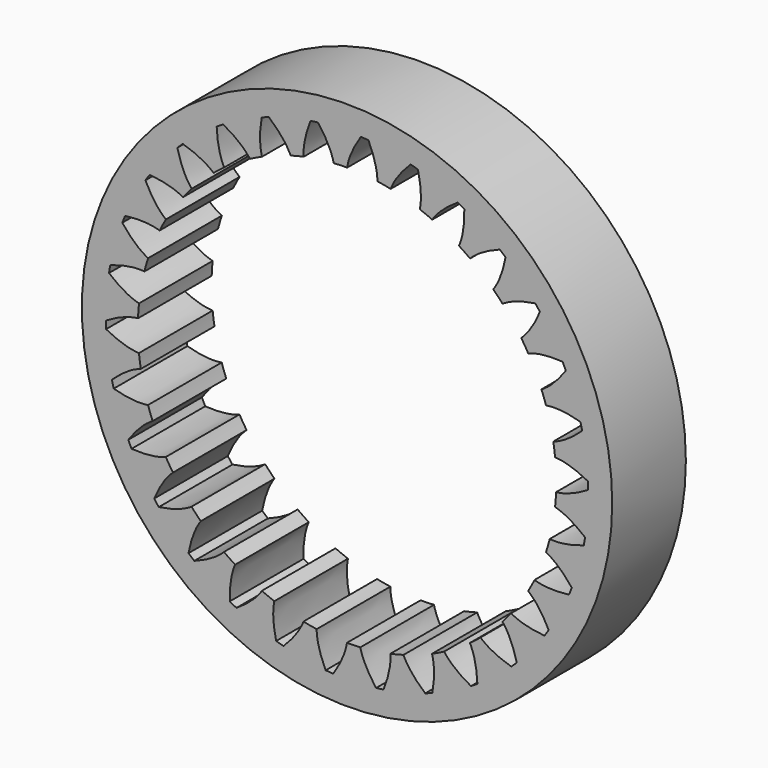
from build123d import *

# Parameters (mm, degrees)
F0_R            = 14.4
F1_DEPTH        = 5
F2_DEPTH        = 5
F2_COPIES_COUNT = 30


# Not quite as in the source:
# - a pattern or mirror of a feature is missing from the dataset's text; its kind, count and spacing are read off the source's solid


with BuildPart() as f1:
    # F0 (on Front) → F1 (new body)
    with BuildSketch(Plane.XZ):
        Circle(F0_R)
        with BuildLine():
            ThreePointArc((-1.576958744, 13.0047376413), (-0.4143593333, 13.0934451671), (0.7515226609, 13.078425505))
            ThreePointArc((0.7515226609, 13.078425505), (9.5250970299, 8.9934713304), (13.1, 0))
            ThreePointArc((13.1, 0), (-8.6876878528, -9.8047988135), (-1.576958744, 13.0047376413))
        make_face(mode=Mode.SUBTRACT)
    extrude(amount=F1_DEPTH)

    # F0 (on Front) → F2 (join)
    with BuildSketch(Plane.XZ):
        with BuildLine():
            add(Edge.make_bspline(
                [(0.7515226609, 13.078425505), (0.668846025, 12.9566216673), (0.4313184402, 12.5782753702), (0.1483402589, 11.9774798358), (0.0327695887, 11.5399474206), (0.0100057071, 11.3857140571), (0.0068165354, 11.3599979549)],
                knots=[0.2131057161, 0.2131057161, 0.2131057161, 0.2131057161, 0.3474795918, 0.6411546656, 0.8686378249, 0.9222849289, 0.9222849289, 0.9222849289, 0.9222849289], degree=3))
            ThreePointArc((0.7515226609, 13.078425505), (-0.4143593333, 13.0934451671), (-1.576958744, 13.0047376413))
            add(Edge.make_bspline(
                [(-1.576958744, 13.0047376413), (-1.486745969, 12.8884051169), (-1.2257710945, 12.5258345874), (-0.9053712565, 11.9441337458), (-0.7623669662, 11.5147842761), (-0.7298965649, 11.3622988743), (-0.7250877632, 11.3368358785)],
                knots=[0.2131057161, 0.2131057161, 0.2131057161, 0.2131057161, 0.3474795918, 0.6411546656, 0.8686378249, 0.9222849289, 0.9222849289, 0.9222849289, 0.9222849289], degree=3))
            ThreePointArc((-0.7250877632, 11.3368358785), (-0.3593222921, 11.354315809), (0.0068165354, 11.3599979549))
        make_face()
    f2 = extrude(amount=F2_DEPTH)

    # F2_copies: F2 ×30 about axis
    f2_copies_axis = Axis((0, 0, 0), (0, 1, 0))
    for i in range(1, F2_COPIES_COUNT):
        add(f2.rotate(f2_copies_axis, i * 360 / F2_COPIES_COUNT))


solid = f1.part
